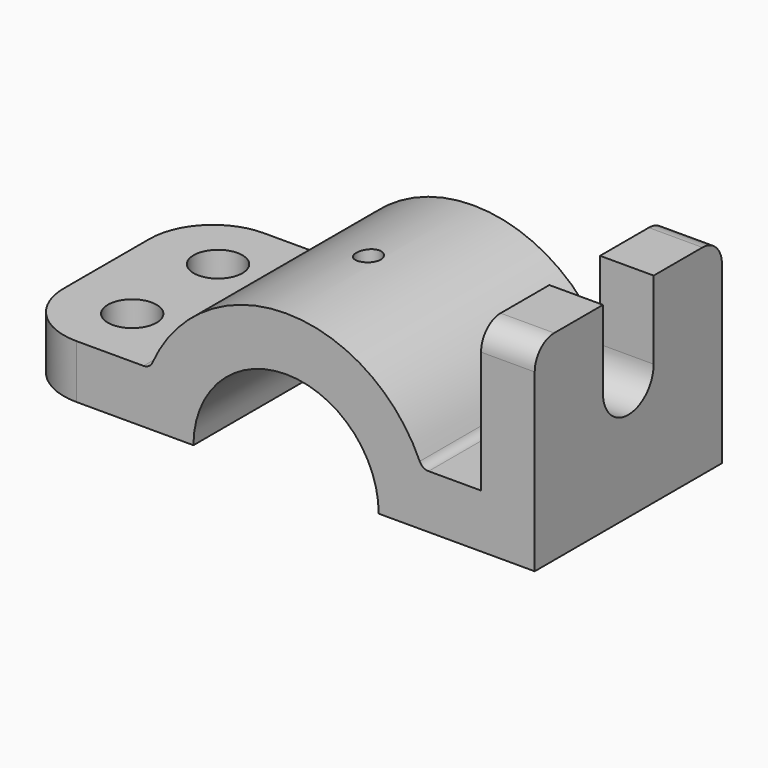
from build123d import *

# Parameters (mm, degrees)
F0_W     = 11
F0_H     = 30
F1_DEPTH = 24
F3_DEPTH = 25
F4_R     = 5
F4_R_2   = 2.5
F5_DEPTH = 25
F6_R     = 13
F7_R     = 5
F8_R     = 2


with BuildPart() as f1:
    # F0 (on Front) → F1 (new body, symmetric)
    with BuildSketch(Plane.XZ):
        with BuildLine():
            ThreePointArc((-27.6980438828, -19.9313075026), (-27.1710581859, -14.3329659721), (-25.6086153568, -8.9313075026))
            Line((-25.6086153568, -8.9313075026), (-53.6980438828, -8.9313075026))
            Line((-53.6980438828, -8.9313075026), (-53.6980438828, -19.9313075026))
            Line((-53.6980438828, -19.9313075026), (-27.6980438828, -19.9313075026))
        make_face()
        with BuildLine():
            Line((-13.1899772677, -8.9313075026), (-25.6086153568, -8.9313075026))
            ThreePointArc((-25.6086153568, -8.9313075026), (-27.1710581859, -14.3329659721), (-27.6980438828, -19.9313075026))
            Line((-27.6980438828, -19.9313075026), (-16.6980438828, -19.9313075026))
            ThreePointArc((-16.6980438828, -19.9313075026), (-15.7997942721, -14.1583851192), (-13.1899772677, -8.9313075026))
        make_face()
        with BuildLine():
            Line((17.793889502, -8.9313075026), (30.2125275911, -8.9313075026))
            ThreePointArc((30.2125275911, -8.9313075026), (2.3019561172, 10.0686924974), (-25.6086153568, -8.9313075026))
            Line((-25.6086153568, -8.9313075026), (-13.1899772677, -8.9313075026))
            ThreePointArc((-13.1899772677, -8.9313075026), (2.3019561172, -0.9313075026), (17.793889502, -8.9313075026))
        make_face()
        with BuildLine():
            ThreePointArc((32.3019561172, -19.9313075026), (31.7749704202, -14.3329659721), (30.2125275911, -8.9313075026))
            Line((30.2125275911, -8.9313075026), (17.793889502, -8.9313075026))
            ThreePointArc((17.793889502, -8.9313075026), (20.4037065064, -14.1583851192), (21.3019561172, -19.9313075026))
            Line((21.3019561172, -19.9313075026), (32.3019561172, -19.9313075026))
        make_face()
        with BuildLine():
            Line((53.3019561172, -8.9313075026), (42.3019561172, -8.9313075026))
            Line((42.3019561172, -8.9313075026), (30.2125275911, -8.9313075026))
            ThreePointArc((30.2125275911, -8.9313075026), (31.7749704202, -14.3329659721), (32.3019561172, -19.9313075026))
            Line((32.3019561172, -19.9313075026), (53.3019561172, -19.9313075026))
            Line((53.3019561172, -19.9313075026), (53.3019561172, -8.9313075026))
        make_face()
        with Locations((47.8019561172, 6.0686924974)):
            Rectangle(F0_W, F0_H)
    extrude(amount=F1_DEPTH, both=True)

    # F2 (on face) → F3 (cut)
    with BuildSketch(Plane.YZ.offset(53.3019561172)):
        with BuildLine():
            ThreePointArc((-6.5, 5.0686926821), (-9.23e-08, -1.4313075026), (6.5, 5.0686924974))
            ThreePointArc((6.5, 5.0686924974), (9.23e-08, 11.5686924974), (-6.5, 5.0686926821))
        make_face()
        with BuildLine():
            ThreePointArc((-6.5, 5.0686926821), (9.23e-08, 11.5686924974), (6.5, 5.0686924974))
            Line((6.5, 5.0686924974), (6.5, 21.0686924974))
            Line((6.5, 21.0686924974), (-6.5, 21.0686924974))
            Line((-6.5, 21.0686924974), (-6.5, 5.0686926821))
        make_face()
    extrude(amount=-F3_DEPTH, mode=Mode.SUBTRACT)

    # F4 (on face) → F5 (cut, symmetric)
    with BuildSketch(Plane.XY.offset(-8.9313075026)):
        with Locations((-39.6533296198, -11)):
            Circle(F4_R)
        with Locations((-39.6533296198, 11)):
            Circle(F4_R)
        Circle(F4_R_2)
    extrude(amount=F5_DEPTH, both=True, mode=Mode.SUBTRACT)

    # F6
    f6_edges = [f1.edges().sort_by_distance(p)[0] for p in [
        (-53.698044, 24, -14.431308),
        (-53.698044, -24, -14.431308),
    ]]
    fillet(f6_edges, radius=F6_R)

    # F7
    f7_edges = [f1.edges().sort_by_distance(p)[0] for p in [
        (47.801956, 24, 21.068692),
        (47.801956, -24, 21.068692),
    ]]
    fillet(f7_edges, radius=F7_R)

    # F8
    f8_edges = [f1.edges().sort_by_distance(p)[0] for p in [
        (30.212528, 0, -8.931308),
        (-25.608615, 0, -8.931308),
    ]]
    fillet(f8_edges, radius=F8_R)


solid = f1.part
